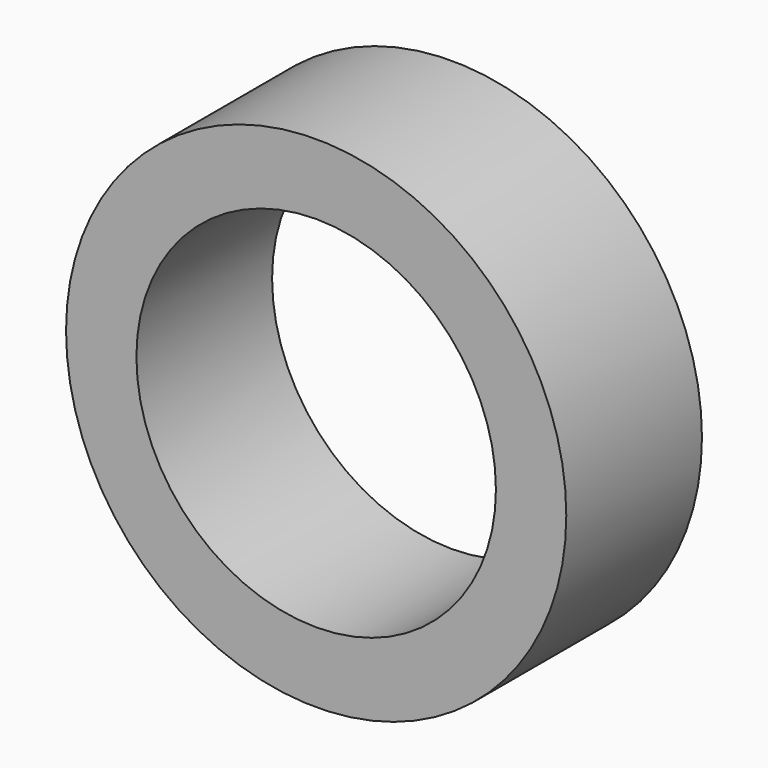
from build123d import *

# Parameters (mm, degrees)
F0_R     = 37.465
F0_R_2   = 26.924
F1_DEPTH = 25.4


# Not quite as in the source:
# - a feature of the source that left no trace in its solid (it failed there, or was rolled back) is left out


with BuildPart() as f1:
    # F0 (on Front) → F1 (new body)
    with BuildSketch(Plane.XZ):
        Circle(F0_R)
        Circle(F0_R_2, mode=Mode.SUBTRACT)
    extrude(amount=F1_DEPTH)


solid = f1.part
